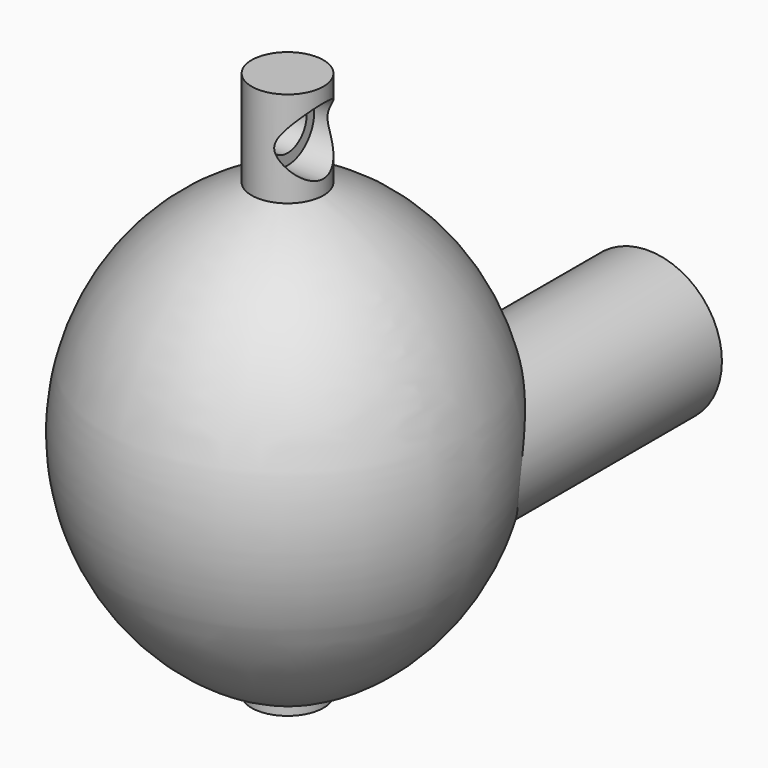
from build123d import *

# Parameters (mm, degrees)
F4_R      = 3.6618559104
F5_DEPTH  = 16.256
F6_R      = 1.7816904606
F7_DEPTH  = 27.178
F8_R      = 1.1877343137
F9_DEPTH  = 72.136
F10_R     = 1.6542577125
F11_DEPTH = 132.588


# Not quite as in the source:
# - the program builds the solid bodies; features that only make, move or delete a surface that nothing else refers to are left out


with BuildPart() as f1:
    # F0 (on Front) → F1 (revolve)
    with BuildSketch(Plane.XZ):
        with BuildLine():
            Line((0, 22.9268427938), (0, 0))
            ThreePointArc((0, 0), (9.3672569036, 11.4634213969), (0, 22.9268427938))
        make_face()
    revolve(axis=Axis((0, 0, 11.4634213969), (0, 0, 1)))

    # F4 (on Front) → F5 (join)
    with BuildSketch(Plane.XZ):
        with Locations((4.9128951505, 10.7615785673)):
            Circle(F4_R)
    extrude(amount=-F5_DEPTH)

    # F6 (on Top) → F7 (join)
    with BuildSketch(Plane.XY):
        Circle(F6_R)
    extrude(amount=F7_DEPTH)

    # F8 (on Right) → F9 (cut)
    with BuildSketch(Plane.YZ):
        with Locations((0, 24.8752553016)):
            Circle(F8_R)
    extrude(amount=-F9_DEPTH, mode=Mode.SUBTRACT)

    # F10 (on Right) → F11 (cut)
    with BuildSketch(Plane.YZ):
        with Locations((0, 24.7984230518)):
            Circle(F10_R)
    extrude(amount=F11_DEPTH, mode=Mode.SUBTRACT)


solid = f1.part
